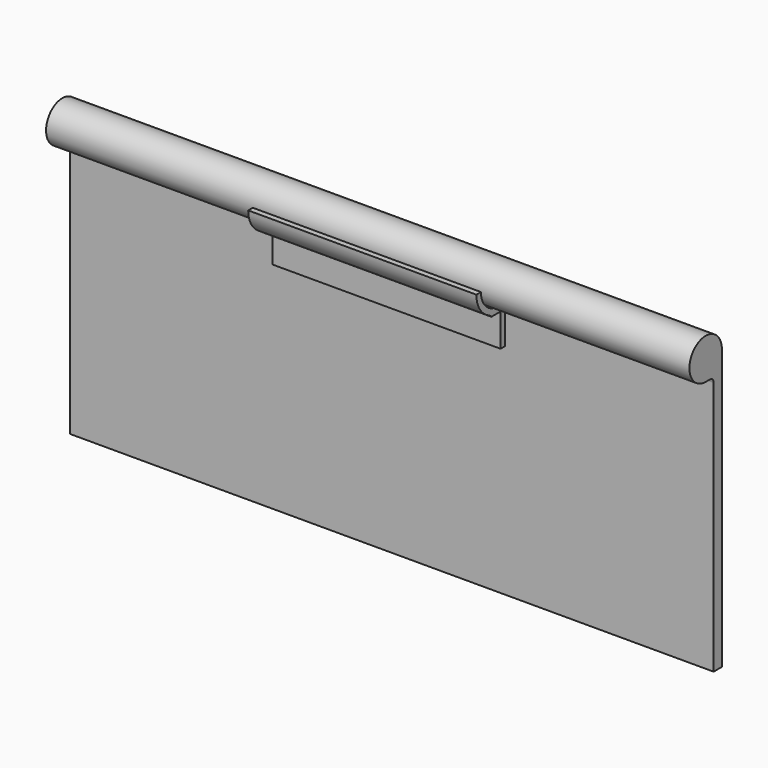
from build123d import *

# Parameters (mm, degrees)
F1_DEPTH    = 141
F3_DEPTH    = 50
F4_T1_DEPTH = 100


# Not quite as in the source:
# - a fillet or chamfer that OpenCascade refuses, or shapes differently, is made with other operations: its cross-section is extruded or revolved along the edge and cut away or added


with BuildPart() as f1:
    # F0 (on Right) → F1 (new body, symmetric)
    with BuildSketch(Plane.YZ):
        with BuildLine():
            ThreePointArc((0, -8.9), (6.2932503526, -6.2932503526), (8.9, 0))
            ThreePointArc((8.9, 0), (-6.2932503526, 6.2932503526), (0, -8.9))
        make_face()
        with BuildLine():
            Line((8.9, -122.5), (8.9, 0))
            ThreePointArc((8.9, 0), (6.2932503526, -6.2932503526), (0, -8.9))
            Line((0, -8.9), (2.35, -8.9))
            ThreePointArc((2.35, -8.9), (3.7642135624, -9.4857864376), (4.35, -10.9))
            Line((4.35, -10.9), (4.35, -122.5))
            Line((4.35, -122.5), (8.9, -122.5))
        make_face()
    extrude(amount=F1_DEPTH, both=True)


with BuildPart() as f3:
    # F2 (on Right) → F3 (new body, symmetric)
    with BuildSketch(Plane.YZ):
        with BuildLine():
            ThreePointArc((0, -9.4), (-6.6468037432, -6.6468037432), (-9.4, 0))
            Line((-9.4, 0), (-11.9, 0))
            ThreePointArc((-11.9, 0), (-9.618861679, -7.0062472123), (-3.65, -11.3264071973))
            ThreePointArc((-3.65, -11.3264071973), (-1.8473974259, -11.7557272319), (-4.02e-08, -11.9))
            ThreePointArc((-4.02e-08, -11.9), (0.6760920348, -11.8807785755), (1.35, -11.8231763922))
            ThreePointArc((1.35, -11.8231763922), (2.6127340162, -11.6096348332), (3.8452078973, -11.2616329289))
            ThreePointArc((3.8452078973, -11.2616329289), (3.2144166992, -9.9376843463), (1.85, -9.4))
            Line((1.85, -9.4), (0, -9.4))
        make_face()
        with BuildLine():
            ThreePointArc((-4.02e-08, -11.9), (-1.8473974259, -11.7557272319), (-3.65, -11.3264071973))
            Line((-3.65, -11.3264071973), (-3.65, -11.9))
            Line((-3.65, -11.9), (-4.02e-08, -11.9))
        make_face()
        with BuildLine():
            ThreePointArc((3.85, -11.4), (3.8488016153, -11.3307749854), (3.8452078973, -11.2616329289))
            ThreePointArc((3.8452078973, -11.2616329289), (2.6127340162, -11.6096348332), (1.35, -11.8231763922))
            Line((1.35, -11.8231763922), (1.35, -11.9))
            Line((1.35, -11.9), (1.35, -26.2599955595))
            Line((1.35, -26.2599955595), (3.85, -26.2599955595))
            Line((3.85, -26.2599955595), (3.85, -11.4))
        make_face()
        with BuildLine():
            ThreePointArc((3.85, -11.2599955595), (3.8476040358, -11.2608144991), (3.8452078973, -11.2616329289))
            ThreePointArc((3.8452078973, -11.2616329289), (3.8488016153, -11.3307749854), (3.85, -11.4))
            Line((3.85, -11.4), (3.85, -11.2599955595))
        make_face()
        with BuildLine():
            ThreePointArc((1.35, -11.8231763922), (0.6760920348, -11.8807785755), (-4.02e-08, -11.9))
            Line((-4.02e-08, -11.9), (1.35, -11.9))
            Line((1.35, -11.9), (1.35, -11.8231763922))
        make_face()
    extrude(amount=F3_DEPTH, both=True)

    # F4: fillet of radius 5 on 1 edges, made by hand

    # F4_s2 → F4_t1 (join)
    with BuildSketch(Plane.YZ.offset(-50)):
        with BuildLine():
            ThreePointArc((-3.65, -11.9), (-4.3769843949, -11.2167783036), (-5.2251400827, -10.6914877878))
            ThreePointArc((-5.2251400827, -10.6914877878), (-4.4489109382, -11.0370825612), (-3.65, -11.3264071973))
            Line((-3.65, -11.3264071973), (-3.65, -11.9))
        make_face()
    extrude(amount=F4_T1_DEPTH)


solid = Compound([f1.part, f3.part])
